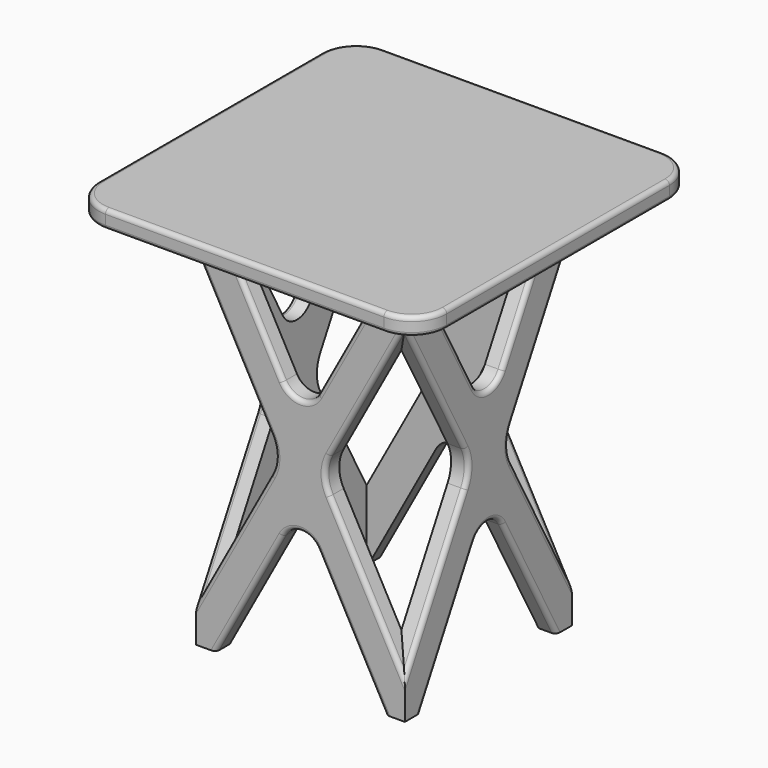
from build123d import *

# Parameters (mm, degrees)
F1_START = 127
F1_DEPTH = 25.4
F2_SIZE  = 25.39999
F3_R     = 6.35
F4_COUNT = 4
F5_W     = 508
F5_H     = 508
F6_DEPTH = 25.4
F7_R     = 50.8
F8_R     = 6.35
F9_R     = 5.08


# Not quite as in the source:
# - a fillet or chamfer is up to 0.001 mm smaller than in the source, because OpenCascade refuses the exact size
# - ends of sketch curves that miss each other by under 0.0002 mm in the source are joined


with BuildPart() as f1:
    # F0 (on Right) → F1 (new body)
    with BuildSketch(Plane.YZ.offset(F1_START)):
        with BuildLine():
            Line((-123.4671738375, 558.8), (-152.4, 558.8))
            Line((-152.4, 558.8), (-152.4, 505.7564853687))
            Line((-152.4, 505.7564853687), (-42.7873716171, 304.8))
            ThreePointArc((-42.7873716171, 304.8), (-36.3105236524, 279.4), (-42.7873716171, 254))
            Line((-42.7873716171, 254), (-152.4, 53.0435146313))
            Line((-152.4, 53.0435146313), (-152.4, 0))
            Line((-152.4, 0), (-123.4671738375, 0))
            Line((-123.4671738375, 0), (-25.4, 179.789818702))
            ThreePointArc((-25.4, 179.789818702), (0, 194.86809941), (25.4, 179.789818702))
            Line((25.4, 179.789818702), (123.4671738375, 0))
            Line((123.4671738375, 0), (152.4, 0))
            Line((152.4, 0), (152.4, 53.0435146313))
            Line((152.4, 53.0435146313), (42.7873716171, 254))
            ThreePointArc((42.7873716171, 254), (36.3105236524, 279.4), (42.7873716171, 304.8))
            Line((42.7873716171, 304.8), (152.4, 505.7564853687))
            Line((152.4, 505.7564853687), (152.4, 558.8))
            Line((152.4, 558.8), (123.4671738375, 558.8))
            Line((123.4671738375, 558.8), (25.4, 379.010181298))
            ThreePointArc((25.4, 379.010181298), (0, 363.93190059), (-25.4, 379.010181298))
            Line((-25.4, 379.010181298), (-123.4671738375, 558.8))
        make_face()
    extrude(amount=F1_DEPTH)

    # F2 (size 25.4 in the source; OpenCascade refuses exactly that, so slightly less here)
    f2_edges = [f1.edges().sort_by_distance(p)[0] for p in [
        (127, 152.4, 532.278243),
        (127, 152.4, 26.521757),
        (127, -152.4, 532.278243),
        (127, -152.4, 26.521757),
    ]]
    chamfer(f2_edges, length=F2_SIZE)

    # F3
    f3_edges = [f1.edges().sort_by_distance(p)[0] for p in [
        (152.4, -97.593686, 405.278243),
        (152.4, -74.433587, 468.905091),
        (152.4, 97.593686, 405.278243),
        (152.4, 74.433587, 89.894909),
    ]]
    fillet(f3_edges, radius=F3_R)


with BuildPart() as f4_1:
    # F4: instance of F1
    add(f1.part.rotate(Axis((0, 0, 279.4), (0, 0, 1)), 1 * 360 / F4_COUNT))


with BuildPart() as f4_2:
    # F4: instance of F1
    add(f1.part.rotate(Axis((0, 0, 279.4), (0, 0, 1)), 2 * 360 / F4_COUNT))


with BuildPart() as f4_3:
    # F4: instance of F1
    add(f1.part.rotate(Axis((0, 0, 279.4), (0, 0, 1)), 3 * 360 / F4_COUNT))


with BuildPart() as f6:
    # F5 (on face) → F6 (new body)
    with BuildSketch(Plane.XY.offset(558.8)):
        Rectangle(F5_W, F5_H)
        with BuildLine():
            Line((152.4, 152.4), (152.4, 130.7003803781))
            add(Edge.make_bspline(
                [(152.4, 130.7003803781), (152.4, 123.4671738375), (146.05, 123.4671738375)],
                knots=[4.7123889804, 4.7123889804, 4.7123889804, 6.2831853072, 6.2831853072, 6.2831853072], degree=2, weights=[1, 0.7071067812, 1]))
            Line((146.05, 123.4671738375), (127, 123.4671738375))
            Line((127, 123.4671738375), (127, 127.00001))
            Line((127, 127.00001), (152.4, 152.4))
        make_face(mode=Mode.SUBTRACT)
        with BuildLine():
            add(Edge.make_bspline(
                [(152.4, 130.7003803781), (152.4, 123.4671738375), (146.05, 123.4671738375)],
                knots=[4.7123889804, 4.7123889804, 4.7123889804, 6.2831853072, 6.2831853072, 6.2831853072], degree=2, weights=[1, 0.7071067812, 1]))
            Line((152.4, 130.7003803781), (152.4, 152.4))
            Line((152.4, 152.4), (127, 127.00001))
            Line((127, 127.00001), (127, 123.4671738375))
            Line((127, 123.4671738375), (146.05, 123.4671738375))
        make_face()
    extrude(amount=F6_DEPTH)

    # F7
    f7_edges = [f6.edges().sort_by_distance(p)[0] for p in [
        (-254, 254, 571.5),
        (-254, -254, 571.5),
        (254, 254, 571.5),
        (254, -254, 571.5),
    ]]
    fillet(f7_edges, radius=F7_R)

    # F8
    f8_edges = [f6.edges().sort_by_distance(p)[0] for p in [
        (0, -254, 584.2),
    ]]
    fillet(f8_edges, radius=F8_R)

    # F9
    f9_edges = [f6.edges().sort_by_distance(p)[0] for p in [
        (0, -254, 558.8),
    ]]
    fillet(f9_edges, radius=F9_R)


solid = Compound([f1.part, f4_1.part, f4_2.part, f4_3.part, f6.part])
